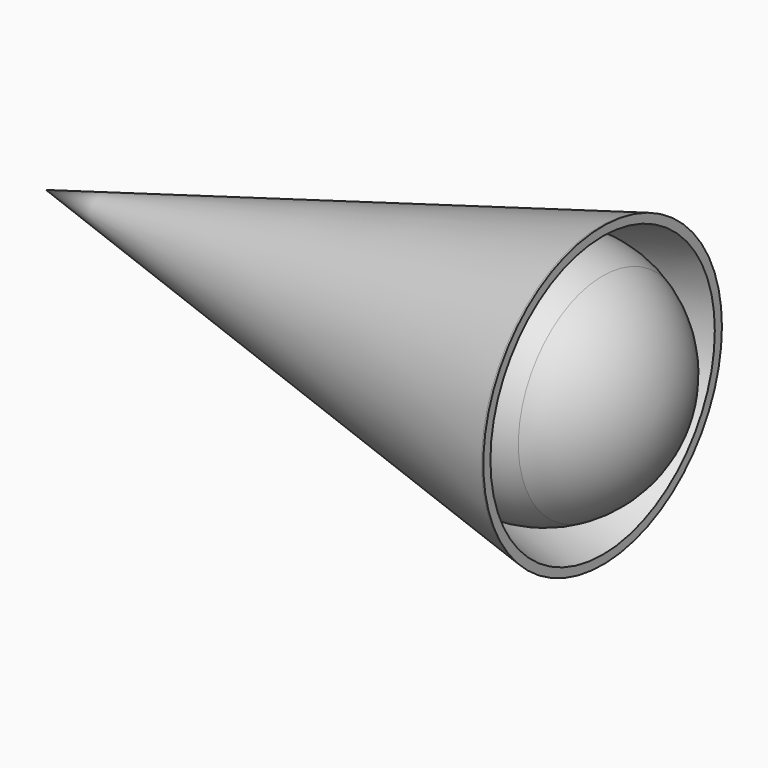
from build123d import *


with BuildPart() as f1:
    # F0 (on Top) → F1 (revolve)
    with BuildSketch(Plane.XY):
        with BuildLine():
            Line((-70.104, 0), (33.9389434953, 0))
            Line((33.9389434953, 0), (33.9389434953, 61.3410052935))
            ThreePointArc((33.9389434953, 61.3410052935), (8.5162125913, 69.5848039381), (-18.1442503379, 67.7152641262))
            ThreePointArc((-18.1442503379, 67.7152641262), (-55.6172425678, 42.6766112192), (-70.104, 0))
        make_face()
    revolve(axis=Axis((-118.4610565047, 0, 0), (-1, 0, 0)))

    # F0 (on Top) → F2 (revolve)
    with BuildSketch(Plane.XY):
        with BuildLine():
            Line((33.9389434953, 61.3410052935), (33.9389434953, 0))
            Line((33.9389434953, 0), (70.104, 0))
            ThreePointArc((70.104, 0), (60.3896783846, 35.6041789767), (33.9389434953, 61.3410052935))
        make_face()
    revolve(axis=Axis((-118.4610565047, 0, 0), (-1, 0, 0)))

    # F0 (on Top) → F3 (revolve)
    with BuildSketch(Plane.XY):
        Polygon((-18.1442503379, 67.7152641262), (33.9389434953, 81.670913853), (33.9389434953, 86.8472932512), (32.6448486458, 86.5005415813), (-272.1551513542, 4.8296277283), (-290.1795674178, 0), (-270.8610565047, 0), align=None)
    revolve(axis=Axis((-118.4610565047, 0, 0), (-1, 0, 0)))

    # F0 (on Top) → F4 (revolve)
    with BuildSketch(Plane.XY):
        with BuildLine():
            Line((-270.8610565047, 0), (-70.104, 0))
            ThreePointArc((-70.104, 0), (-55.6172425678, 42.6766112192), (-18.1442503379, 67.7152641262))
            Line((-18.1442503379, 67.7152641262), (-270.8610565047, 0))
        make_face()
    revolve(axis=Axis((-118.4610565047, 0, 0), (-1, 0, 0)))


solid = f1.part
